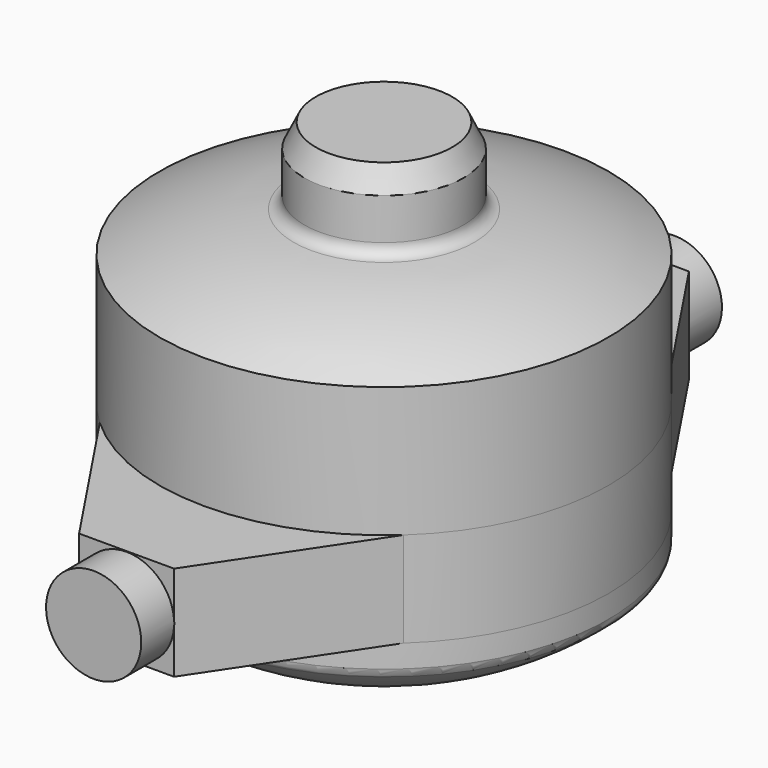
from build123d import *

# Parameters (mm, degrees)
F2_W     = 387.35
F2_H     = 25.4
F6_DEPTH = 25.4


with BuildPart() as f1:
    # F0 (on Right) → F1 (revolve)
    with BuildSketch(Plane.YZ):
        with BuildLine():
            Line((0, -118.26875), (0, 118.26875))
            Line((0, 118.26875), (-36.4434868097, 118.26875))
            Line((-36.4434868097, 118.26875), (-42.4832068384, 105.8115510884))
            Line((-42.4832068384, 105.8115510884), (-42.4832068384, 83.7009549141))
            ThreePointArc((-42.4832068384, 83.7009549141), (-44.1215808782, 79.4438337258), (-48.1912637869, 77.3834863452))
            ThreePointArc((-48.1912637869, 77.3834863452), (-85.0232586464, 70.1110976422), (-119.85625, 56.1058773246))
            Line((-119.85625, 56.1058773246), (-119.85625, -76.3638510721))
            ThreePointArc((-119.85625, -76.3638510721), (-119.2664236189, -79.0364714867), (-117.6065177542, -81.212593625))
            ThreePointArc((-117.6065177542, -81.212593625), (-62.5274204439, -111.5601835015), (0, -118.26875))
        make_face()
    revolve(axis=Axis((0, 0, 0), (0, 0, -1)))

    # F2 (on Right) → F3 (revolve)
    with BuildSketch(Plane.YZ):
        with Locations((0, -26.5370635647)):
            Rectangle(F2_W, F2_H)
    revolve(axis=Axis((0, 0, -39.2370635647), (0, 1, 0)))

    # F5 (on offset) → F6 (join, symmetric)
    with BuildSketch(Plane.XY.offset(-38.8874)):
        with BuildLine():
            Line((25.3370366991, 171.7288643122), (0, 171.7288643122))
            Line((0, 171.7288643122), (-25.3370366991, 171.7288643122))
            Line((-25.3370366991, 171.7288643122), (-81.0122731187, 88.3319436456))
            ThreePointArc((-81.0122731187, 88.3319436456), (-119.85625, 0), (-81.0122731187, -88.3319436456))
            Line((-81.0122731187, -88.3319436456), (-25.3370366991, -171.7288643122))
            Line((-25.3370366991, -171.7288643122), (0, -171.7288643122))
            Line((0, -171.7288643122), (25.3370366991, -171.7288643122))
            Line((25.3370366991, -171.7288643122), (81.0122731187, -88.3319436456))
            ThreePointArc((81.0122731187, -88.3319436456), (119.85625, 0), (81.0122731187, 88.3319436456))
            Line((81.0122731187, 88.3319436456), (25.3370366991, 171.7288643122))
        make_face()
    extrude(amount=F6_DEPTH, both=True)


solid = f1.part
